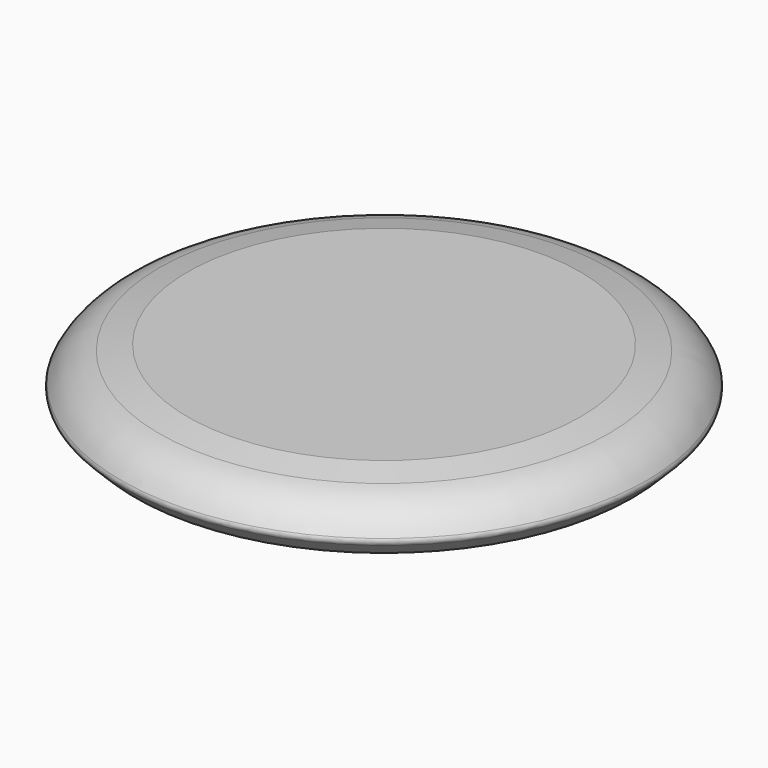
from build123d import *

# Parameters (mm, degrees)
F2_SIZE = 7.62
F4_R    = 2.54
F5_R    = 5.08


# Not quite as in the source:
# - a fillet or chamfer that OpenCascade refuses, or shapes differently, is made with other operations: its cross-section is extruded or revolved along the edge and cut away or added


with BuildPart() as f1:
    # F0 (on Front) → F1 (revolve)
    with BuildSketch(Plane.XZ):
        Polygon((89.2264246941, 28.6549665034), (0, 28.6549665034), (0, 22.5978214294), (89.2264246941, 22.5978214294), (106.4660027623, 16.5406726301), (106.4660027623, 3.9604459889), (120.4440295696, 3.9604459889), (120.4440295696, 22.5978214294), align=None)
    revolve(axis=Axis((0, 0, 25.6263939664), (0, 0, 1)))

    # F2
    f2_edges = [f1.edges().sort_by_distance(p)[0] for p in [
        (-120.44403, 0, 3.960446),
    ]]
    chamfer(f2_edges, length=F2_SIZE)

    # F3: fillet of radius 25.4 on 1 edges, made by hand

    # F3_s1 → F3_t2 (revolve, cut)
    with BuildSketch(Plane.XZ):
        with BuildLine():
            ThreePointArc((120.4440295696, 11.5804459889), (113.0489234012, 21.1136915786), (102.0892995141, 26.1591857039))
            Line((102.0892995141, 26.1591857039), (120.4440295696, 22.5978214294))
            Line((120.4440295696, 22.5978214294), (120.4440295696, 11.5804459889))
        make_face()
    revolve(axis=Axis((0, 0, 22.5978214294), (0, 0, 1)), mode=Mode.SUBTRACT)

    # F4
    f4_edges = [f1.edges().sort_by_distance(p)[0] for p in [
        (-120.44403, 0, 11.580446),
    ]]
    fillet(f4_edges, radius=F4_R)

    # F5
    f5_edges = [f1.edges().sort_by_distance(p)[0] for p in [
        (-106.466003, 0, 16.540673),
    ]]
    fillet(f5_edges, radius=F5_R)


solid = f1.part
